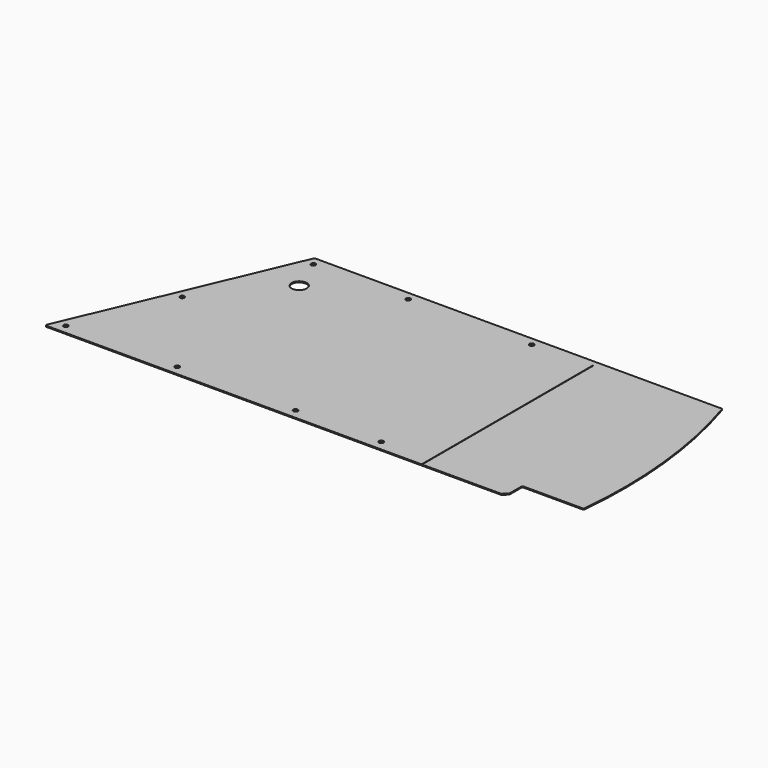
from build123d import *

# Parameters (mm, degrees)
F1_DEPTH = 3
F2_SIZE  = 9.525
F4_DEPTH = 0.7493
F6_D     = 9.525
F8_D     = 31.75
F9_R     = 2.54


# Not quite as in the source:
# - a length typed as a fraction of an inch, garbled in the dataset ("3 / 203.2 mm" for 3/8 in), is restored


with BuildPart() as f1:
    # F0 (on Top) → F1 (new body)
    with BuildSketch(Plane.XY):
        with BuildLine():
            Line((197.5066929404, 463.55), (0, 0))
            Line((0, 0), (971.55, 0))
            Line((971.55, 0), (971.55, 43.18))
            Line((971.55, 43.18), (1101.00364, 43.18))
            ThreePointArc((1101.00364, 43.18), (1100.0520555905, 255.6158899642), (1056.5397729404, 463.55))
            Line((1056.5397729404, 463.55), (197.5066929404, 463.55))
        make_face()
    extrude(amount=F1_DEPTH)

    # F2
    f2_edges = [f1.edges().sort_by_distance(p)[0] for p in [
        (971.55, 0, 1.5),
    ]]
    chamfer(f2_edges, length=F2_SIZE)

    # F3 (on face) → F4 (cut)
    with BuildSketch(Plane.XY.offset(3)):
        with BuildLine():
            Line((0, 0), (793.26486, 0))
            Line((793.26486, 0), (793.26486, 451.36562))
            Line((793.26486, 451.36562), (794.85236, 451.36562))
            Line((794.85236, 451.36562), (794.85236, 0))
            Line((794.85236, 0), (962.025, 0))
            Line((962.025, 0), (971.55, 9.525))
            Line((971.55, 9.525), (971.55, 43.18))
            Line((971.55, 43.18), (1101.00364, 43.18))
            ThreePointArc((1101.00364, 43.18), (1100.0520555905, 255.6158899642), (1056.5397729404, 463.55))
            Line((1056.5397729404, 463.55), (197.5066929404, 463.55))
            Line((197.5066929404, 463.55), (0, 0))
        make_face()
    extrude(amount=-F4_DEPTH, mode=Mode.SUBTRACT)

    # F6 (through all)
    with Locations(Plane.XY.offset(2.2507)):
        with Locations((209.7413209615, 445.0286267957), (409.2329209615, 445.516), (669.1511209615, 446.151), (113.7415553228, 219.7163059861), (28.5242, 19.7104), (262.7122, 20.176624196), (511.8862, 20.6726826953), (691.9722, 21.0312)):
            Hole(F6_D / 2)

    # F8 (through all)
    with Locations(Plane.XY.offset(2.2507)):
        with Locations((238.9469804498, 371.2718)):
            Hole(F8_D / 2)

    # F9
    f9_edges = [f1.edges().sort_by_distance(p)[0] for p in [
        (197.506693, 463.55, 1.12535),
        (1056.539773, 463.55, 1.12535),
        (1101.00364, 43.18, 1.12535),
        (971.55, 43.18, 1.12535),
        (971.55, 9.525, 1.12535),
        (962.025, 0, 1.12535),
        (0, 0, 1.12535),
    ]]
    fillet(f9_edges, radius=F9_R)


solid = f1.part
